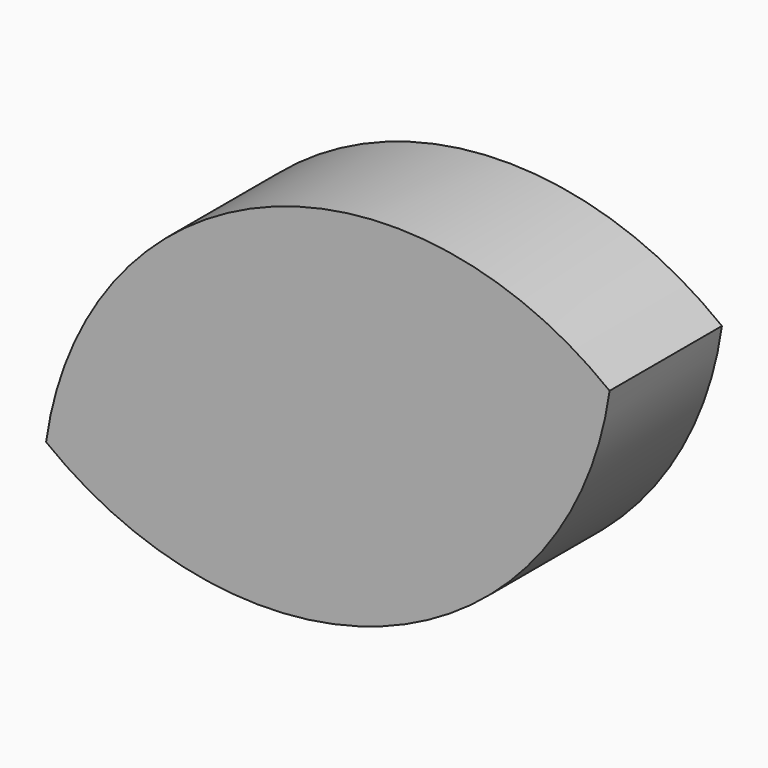
from build123d import *

# Parameters (mm, degrees)
F2_DEPTH = 6


# Not quite as in the source:
# - a feature names something its author has since deleted; it is built from what else it names
# - the program builds the solid bodies; features that only make, move or delete a surface that nothing else refers to are left out


with BuildPart() as f2:
    # F0 (on Front) → F2 (new body)
    with BuildSketch(Plane.XZ):
        with BuildLine():
            ThreePointArc((-55.0104333185, 0), (-40.1542426855, -2.0721003539), (-30.9316558234, 9.7576879608))
            ThreePointArc((-30.9316558234, 9.7576879608), (-45.7878464564, 11.8297883147), (-55.0104333185, 0))
        make_face()
    extrude(amount=F2_DEPTH)


solid = f2.part
